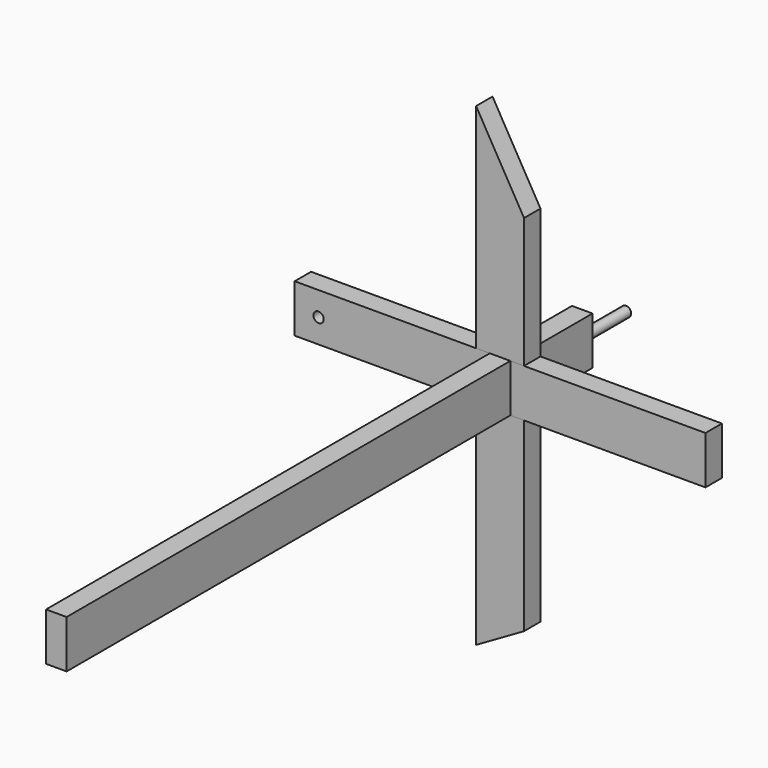
from build123d import *

# Parameters (mm, degrees)
F2_W      = 38.1
F2_H      = 88.9
F3_DEPTH  = 152.4
F5_DEPTH  = 38.1
F6_W      = 762
F6_H      = 88.9
F7_DEPTH  = 38.1
F8_D      = 19.05
F9_R      = 9.525
F10_DEPTH = 254
F11_DEPTH = 1066.8


# Not quite as in the source:
# - a variable given as a bare number and used for a length is read in inches; the dataset says mm whatever the document's units were


with BuildPart() as f3:
    # F2 (on Front) → F3 (new body, symmetric)
    with BuildSketch(Plane.XZ):
        Rectangle(F2_W, F2_H)
    extrude(amount=F3_DEPTH, both=True)


with BuildPart() as f5:
    # F4 (on Front) → F5 (new body)
    with BuildSketch(Plane.XZ):
        Polygon((-44.45, 439.9409051225), (-44.45, -439.9409051225), (44.45, -388.6144661915), (44.45, 285.9615883296), align=None)
    extrude(amount=F5_DEPTH)


with BuildPart() as f7:
    # F6 (on Front) → F7 (new body)
    with BuildSketch(Plane.XZ):
        Rectangle(F6_W, F6_H)
    extrude(amount=F7_DEPTH)

    # F8 (through all)
    with Locations(Plane(origin=(0, 0, 0), x_dir=(1, 0, 0), z_dir=(0, 1, 0))):
        with Locations((-336.55, 0)):
            Hole(F8_D / 2)


with BuildPart() as f10:
    # F9 (on Front) → F10 (new body, symmetric)
    with BuildSketch(Plane.XZ):
        Circle(F9_R)
    extrude(amount=F10_DEPTH, both=True)


with BuildPart() as f11:
    # F2 (on Front) → F11 (new body)
    with BuildSketch(Plane.XZ):
        Rectangle(F2_W, F2_H)
    extrude(amount=F11_DEPTH)


solid = Compound([f3.part, f5.part, f7.part, f10.part, f11.part])
